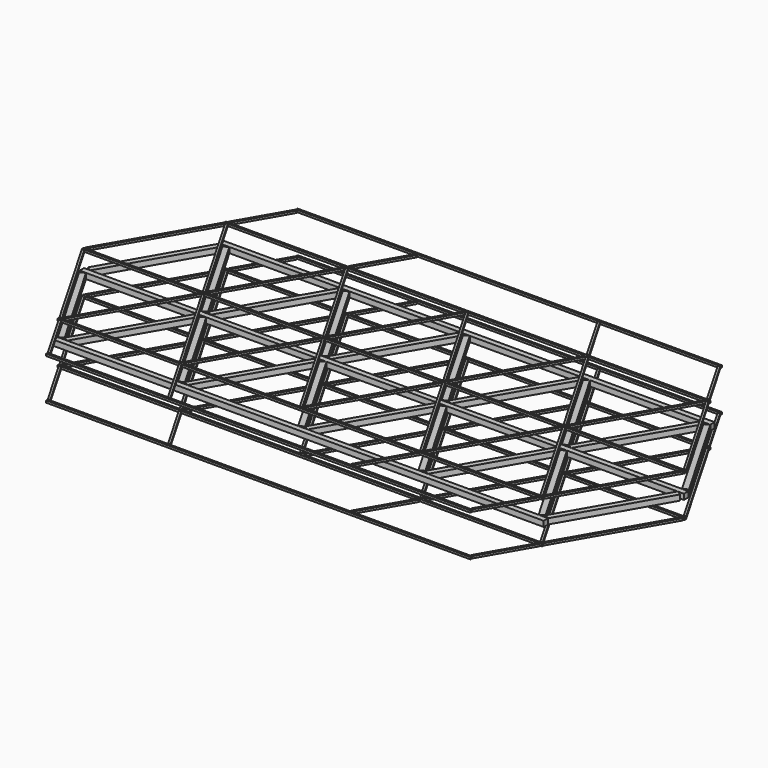
from build123d import *

# Parameters (mm, degrees)
F4_DEPTH = 20
F6_DEPTH = 7.5


# Not quite as in the source:
# - a feature names something its author has since deleted; it is built from what else it names


with BuildPart() as f4:
    # F2 (on Top) → F4 (new body, symmetric)
    with BuildSketch(Plane.XY):
        Polygon((-1789.7858344878, 780), (-1789.7858344878, 740), (-1720.5038021851, 740), (-912.2134253196, 740), (-842.9313930169, 740), (-34.6410161514, 740), (0, 740), (34.6410161514, 740), (842.9313930169, 740), (912.2134253196, 740), (1720.5038021851, 740), (1789.7858344878, 740), (1789.7858344878, 780), (0, 780), align=None)
    extrude(amount=F4_DEPTH, both=True)


with BuildPart() as f4b:
    # F2 (on Top) → F4, piece 2 (new body, symmetric)
    with BuildSketch(Plane.XY):
        Polygon((-2193.9310229206, 40), (-2159.2900067692, 20), (-1755.1448183365, 720), (-1772.4653264122, 730), (-1789.7858344878, 740), align=None)
    extrude(amount=F4_DEPTH, both=True)


with BuildPart() as f4c:
    # F2 (on Top) → F4, piece 3 (new body, symmetric)
    with BuildSketch(Plane.XY):
        Polygon((-1755.1448183365, 720), (-1350.9996299037, 20), (-1333.679121828, 30), (-1316.3586137523, 40), (-1720.5038021851, 740), (-1737.8243102608, 730), align=None)
    extrude(amount=F4_DEPTH, both=True)


with BuildPart() as f4d:
    # F2 (on Top) → F4, piece 4 (new body, symmetric)
    with BuildSketch(Plane.XY):
        Polygon((-1299.0381056767, 30), (-1281.717597601, 20), (-877.5724091682, 720), (-894.8929172439, 730), (-912.2134253196, 740), (-1316.3586137523, 40), align=None)
    extrude(amount=F4_DEPTH, both=True)


with BuildPart() as f4e:
    # F2 (on Top) → F4, piece 5 (new body, symmetric)
    with BuildSketch(Plane.XY):
        Polygon((-877.5724091682, 720), (-473.4272207355, 20), (-456.1067126598, 30), (-438.7862045841, 40), (-842.9313930169, 740), (-860.2519010925, 730), align=None)
    extrude(amount=F4_DEPTH, both=True)


with BuildPart() as f4f:
    # F2 (on Top) → F4, piece 6 (new body, symmetric)
    with BuildSketch(Plane.XY):
        Polygon((-421.4656965084, 30), (-404.1451884327, 20), (0, 720), (-17.3205080757, 730), (-34.6410161514, 740), (-438.7862045841, 40), align=None)
    extrude(amount=F4_DEPTH, both=True)


with BuildPart() as f4g:
    # F2 (on Top) → F4, piece 7 (new body, symmetric)
    with BuildSketch(Plane.XY):
        Polygon((17.3205080757, 730), (0, 720), (404.1451884327, 20), (421.4656965084, 30), (438.7862045841, 40), (34.6410161514, 740), align=None)
    extrude(amount=F4_DEPTH, both=True)


with BuildPart() as f4h:
    # F2 (on Top) → F4, piece 8 (new body, symmetric)
    with BuildSketch(Plane.XY):
        Polygon((456.1067126598, 30), (473.4272207355, 20), (877.5724091682, 720), (860.2519010925, 730), (842.9313930169, 740), (438.7862045841, 40), align=None)
    extrude(amount=F4_DEPTH, both=True)


with BuildPart() as f4i:
    # F2 (on Top) → F4, piece 9 (new body, symmetric)
    with BuildSketch(Plane.XY):
        Polygon((894.8929172439, 730), (877.5724091682, 720), (1281.717597601, 20), (1299.0381056767, 30), (1316.3586137523, 40), (912.2134253196, 740), align=None)
    extrude(amount=F4_DEPTH, both=True)


with BuildPart() as f4j:
    # F2 (on Top) → F4, piece 10 (new body, symmetric)
    with BuildSketch(Plane.XY):
        Polygon((1737.8243102608, 730), (1720.5038021851, 740), (1316.3586137523, 40), (1333.679121828, 30), (1350.9996299037, 20), (1755.1448183365, 720), align=None)
    extrude(amount=F4_DEPTH, both=True)


with BuildPart() as f4k:
    # F2 (on Top) → F4, piece 11 (new body, symmetric)
    with BuildSketch(Plane.XY):
        Polygon((1316.3586137523, -40), (1720.5038021851, -740), (1737.8243102608, -730), (1755.1448183365, -720), (1350.9996299037, -20), (1333.679121828, -30), align=None)
    extrude(amount=F4_DEPTH, both=True)


with BuildPart() as f4l:
    # F2 (on Top) → F4, piece 12 (new body, symmetric)
    with BuildSketch(Plane.XY):
        Polygon((1281.717597601, -20), (877.5724091682, -720), (894.8929172439, -730), (912.2134253196, -740), (1316.3586137523, -40), (1299.0381056767, -30), align=None)
    extrude(amount=F4_DEPTH, both=True)


with BuildPart() as f4m:
    # F2 (on Top) → F4, piece 13 (new body, symmetric)
    with BuildSketch(Plane.XY):
        Polygon((877.5724091682, -720), (473.4272207355, -20), (456.1067126598, -30), (438.7862045841, -40), (842.9313930169, -740), (860.2519010925, -730), align=None)
    extrude(amount=F4_DEPTH, both=True)


with BuildPart() as f4n:
    # F2 (on Top) → F4, piece 14 (new body, symmetric)
    with BuildSketch(Plane.XY):
        Polygon((404.1451884327, -20), (0, -720), (17.3205080757, -730), (34.6410161514, -740), (438.7862045841, -40), (421.4656965084, -30), align=None)
    extrude(amount=F4_DEPTH, both=True)


with BuildPart() as f4o:
    # F2 (on Top) → F4, piece 15 (new body, symmetric)
    with BuildSketch(Plane.XY):
        Polygon((0, -720), (-404.1451884327, -20), (-421.4656965084, -30), (-438.7862045841, -40), (-34.6410161514, -740), (-17.3205080757, -730), align=None)
    extrude(amount=F4_DEPTH, both=True)


with BuildPart() as f4p:
    # F2 (on Top) → F4, piece 16 (new body, symmetric)
    with BuildSketch(Plane.XY):
        Polygon((-456.1067126598, -30), (-473.4272207355, -20), (-877.5724091682, -720), (-860.2519010925, -730), (-842.9313930169, -740), (-438.7862045841, -40), align=None)
    extrude(amount=F4_DEPTH, both=True)


with BuildPart() as f4q:
    # F2 (on Top) → F4, piece 17 (new body, symmetric)
    with BuildSketch(Plane.XY):
        Polygon((-877.5724091682, -720), (-1281.717597601, -20), (-1299.0381056767, -30), (-1316.3586137523, -40), (-912.2134253196, -740), (-894.8929172439, -730), align=None)
    extrude(amount=F4_DEPTH, both=True)


with BuildPart() as f4r:
    # F2 (on Top) → F4, piece 18 (new body, symmetric)
    with BuildSketch(Plane.XY):
        Polygon((-1333.679121828, -30), (-1350.9996299037, -20), (-1755.1448183365, -720), (-1737.8243102608, -730), (-1720.5038021851, -740), (-1316.3586137523, -40), align=None)
    extrude(amount=F4_DEPTH, both=True)


with BuildPart() as f4s:
    # F2 (on Top) → F4, piece 19 (new body, symmetric)
    with BuildSketch(Plane.XY):
        Polygon((-1755.1448183365, -720), (-2159.2900067692, -20), (-2193.9310229206, -40), (-1789.7858344878, -740), (-1772.4653264122, -730), align=None)
    extrude(amount=F4_DEPTH, both=True)


with BuildPart() as f4t:
    # F2 (on Top) → F4, piece 20 (new body, symmetric)
    with BuildSketch(Plane.XY):
        Polygon((-1720.5038021851, -740), (-1789.7858344878, -740), (-1789.7858344878, -780), (0, -780), (1789.7858344878, -780), (1789.7858344878, -740), (1720.5038021851, -740), (912.2134253196, -740), (842.9313930169, -740), (34.6410161514, -740), (0, -740), (-34.6410161514, -740), (-842.9313930169, -740), (-912.2134253196, -740), align=None)
    extrude(amount=F4_DEPTH, both=True)


with BuildPart() as f4u:
    # F2 (on Top) → F4, piece 21 (new body, symmetric)
    with BuildSketch(Plane.XY):
        Polygon((1772.4653264122, -730), (1789.7858344878, -740), (2193.9310229206, -40), (2159.2900067692, -20), (1755.1448183365, -720), align=None)
    extrude(amount=F4_DEPTH, both=True)


with BuildPart() as f4v:
    # F2 (on Top) → F4, piece 22 (new body, symmetric)
    with BuildSketch(Plane.XY):
        Polygon((2193.9310229206, 40), (1789.7858344878, 740), (1772.4653264122, 730), (1755.1448183365, 720), (2159.2900067692, 20), align=None)
    extrude(amount=F4_DEPTH, both=True)


with BuildPart() as f4w:
    # F2 (on Top) → F4, piece 23 (new body, symmetric)
    with BuildSketch(Plane.XY):
        Polygon((-2159.2900067692, 20), (-2205.4780283044, 20), (-2205.4780283044, -20), (-2159.2900067692, -20), (-1350.9996299037, -20), (-1281.717597601, -20), (-473.4272207355, -20), (-404.1451884327, -20), (0, -20), (404.1451884327, -20), (473.4272207355, -20), (1281.717597601, -20), (1350.9996299037, -20), (2159.2900067692, -20), (2205.4780283044, -20), (2205.4780283044, 20), (2159.2900067692, 20), (1350.9996299037, 20), (1281.717597601, 20), (473.4272207355, 20), (404.1451884327, 20), (0, 20), (-404.1451884327, 20), (-473.4272207355, 20), (-1281.717597601, 20), (-1350.9996299037, 20), align=None)
    extrude(amount=F4_DEPTH, both=True)


with BuildPart() as f6:
    # F5 (on offset) → F6 (new body, symmetric)
    with BuildSketch(Plane.XY.offset(150)):
        Polygon((-1329.3489948091, 7.5), (-2180.9406418638, 7.5), (-2198.2611499395, 7.5), (-2198.2611499395, 0), (-2198.2611499395, -7.5), (-2180.9406418638, -7.5), (-1329.3489948091, -7.5), (-1303.3682326956, -7.5), (-451.7765856409, -7.5), (-425.7958235273, -7.5), (0, -7.5), (425.7958235273, -7.5), (451.7765856409, -7.5), (1303.3682326956, -7.5), (1329.3489948091, -7.5), (2180.9406418638, -7.5), (2198.2611499395, -7.5), (2198.2611499395, 0), (2198.2611499395, 7.5), (2180.9406418638, 7.5), (1329.3489948091, 7.5), (1303.3682326956, 7.5), (451.7765856409, 7.5), (425.7958235273, 7.5), (0, 7.5), (-425.7958235273, 7.5), (-451.7765856409, 7.5), (-1303.3682326956, 7.5), align=None)
    extrude(amount=F6_DEPTH, both=True)

    # F5 (on offset) → F6, piece 2 (join, symmetric)
    with BuildSketch(Plane.XY.offset(150)):
        Polygon((-1761.6400088648, 748.75), (-1768.1351993932, 752.5), (-2193.9310229206, 15), (-2187.4358323922, 11.25), (-2180.9406418638, 7.5), (-1755.1448183365, 745), align=None)
    extrude(amount=F6_DEPTH, both=True)

    # F5 (on offset) → F6, piece 3 (join, symmetric)
    with BuildSketch(Plane.XY.offset(150)):
        Polygon((-1316.3586137523, 15), (-1742.1544372797, 752.5), (-1748.6496278081, 748.75), (-1755.1448183365, 745), (-1329.3489948091, 7.5), (-1322.8538042807, 11.25), align=None)
    extrude(amount=F6_DEPTH, both=True)

    # F5 (on offset) → F6, piece 4 (join, symmetric)
    with BuildSketch(Plane.XY.offset(150)):
        Polygon((-884.0675996966, 748.75), (-890.562790225, 752.5), (-1316.3586137523, 15), (-1309.863423224, 11.25), (-1303.3682326956, 7.5), (-877.5724091682, 745), align=None)
    extrude(amount=F6_DEPTH, both=True)

    # F5 (on offset) → F6, piece 5 (join, symmetric)
    with BuildSketch(Plane.XY.offset(150)):
        Polygon((-438.7862045841, 15), (-864.5820281115, 752.5), (-871.0772186398, 748.75), (-877.5724091682, 745), (-451.7765856409, 7.5), (-445.2813951125, 11.25), align=None)
    extrude(amount=F6_DEPTH, both=True)



with BuildPart() as f6b:
    # F5 (on offset) → F6, piece 6 (new body, symmetric)
    with BuildSketch(Plane.XY.offset(150)):
        Polygon((-1535.7517160444, 1125), (-1542.2469065728, 1128.75), (-1548.7420971012, 1132.5), (-1755.1448183365, 775), (-1748.6496278081, 771.25), (-1742.1544372797, 767.5), align=None)
    extrude(amount=F6_DEPTH, both=True)


with BuildPart() as f6_1:
    add(f6.part)

    add(f6b.part)  # F6#7 merges F6b
    # F5 (on offset) → F6, piece 7 (join, symmetric)
    with BuildSketch(Plane.XY.offset(150)):
        Polygon((-864.5820281115, 767.5), (-1742.1544372797, 767.5), (-1768.1351993932, 767.5), (-1768.1351993932, 760), (-1768.1351993932, 752.5), (-1742.1544372797, 752.5), (-890.562790225, 752.5), (-864.5820281115, 752.5), (-12.9903810568, 752.5), (0, 752.5), (12.9903810568, 752.5), (864.5820281115, 752.5), (890.562790225, 752.5), (1742.1544372797, 752.5), (1768.1351993932, 752.5), (1768.1351993932, 760), (1768.1351993932, 767.5), (1742.1544372797, 767.5), (864.5820281115, 767.5), (0, 767.5), align=None)
    extrude(amount=F6_DEPTH, both=True)

    # F5 (on offset) → F6, piece 8 (join, symmetric)
    with BuildSketch(Plane.XY.offset(150)):
        Polygon((-664.6744974046, 1128.75), (-671.1696879329, 1132.5), (-877.5724091682, 775), (-871.0772186398, 771.25), (-864.5820281115, 767.5), (-658.1793068762, 1125), align=None)
    extrude(amount=F6_DEPTH, both=True)

    # F5 (on offset) → F6, piece 9 (join, symmetric)
    with BuildSketch(Plane.XY.offset(150)):
        Polygon((-6.4951905284, 748.75), (-12.9903810568, 752.5), (-438.7862045841, 15), (-432.2910140557, 11.25), (-425.7958235273, 7.5), (0, 745), align=None)
    extrude(amount=F6_DEPTH, both=True)

    # F5 (on offset) → F6, piece 10 (join, symmetric)
    with BuildSketch(Plane.XY.offset(150)):
        Polygon((438.7862045841, 15), (12.9903810568, 752.5), (6.4951905284, 748.75), (0, 745), (425.7958235273, 7.5), (432.2910140557, 11.25), align=None)
    extrude(amount=F6_DEPTH, both=True)

    # F5 (on offset) → F6, piece 11 (join, symmetric)
    with BuildSketch(Plane.XY.offset(150)):
        Polygon((877.5724091682, 775), (671.1696879329, 1132.5), (664.6744974046, 1128.75), (658.1793068762, 1125), (864.5820281115, 767.5), (871.0772186398, 771.25), align=None)
    extrude(amount=F6_DEPTH, both=True)

    # F5 (on offset) → F6, piece 12 (join, symmetric)
    with BuildSketch(Plane.XY.offset(150)):
        Polygon((1755.1448183365, 775), (1548.7420971012, 1132.5), (1542.2469065728, 1128.75), (1535.7517160444, 1125), (1742.1544372797, 767.5), (1748.6496278081, 771.25), align=None)
    extrude(amount=F6_DEPTH, both=True)

    # F5 (on offset) → F6, piece 13 (join, symmetric)
    with BuildSketch(Plane.XY.offset(150)):
        Polygon((1748.6496278081, 748.75), (1742.1544372797, 752.5), (1316.3586137523, 15), (1322.8538042807, 11.25), (1329.3489948091, 7.5), (1755.1448183365, 745), align=None)
    extrude(amount=F6_DEPTH, both=True)

    # F5 (on offset) → F6, piece 14 (join, symmetric)
    with BuildSketch(Plane.XY.offset(150)):
        Polygon((1316.3586137523, 15), (890.562790225, 752.5), (884.0675996966, 748.75), (877.5724091682, 745), (1303.3682326956, 7.5), (1309.863423224, 11.25), align=None)
    extrude(amount=F6_DEPTH, both=True)

    # F5 (on offset) → F6, piece 15 (join, symmetric)
    with BuildSketch(Plane.XY.offset(150)):
        Polygon((871.0772186398, 748.75), (864.5820281115, 752.5), (438.7862045841, 15), (445.2813951125, 11.25), (451.7765856409, 7.5), (877.5724091682, 745), align=None)
    extrude(amount=F6_DEPTH, both=True)

    # F5 (on offset) → F6, piece 16 (join, symmetric)
    with BuildSketch(Plane.XY.offset(150)):
        Polygon((2193.9310229206, 15), (1768.1351993932, 752.5), (1761.6400088648, 748.75), (1755.1448183365, 745), (2180.9406418638, 7.5), (2187.4358323922, 11.25), align=None)
    extrude(amount=F6_DEPTH, both=True)

    # F5 (on offset) → F6, piece 17 (join, symmetric)
    with BuildSketch(Plane.XY.offset(150)):
        Polygon((-1548.7420971012, 1140), (-1548.7420971012, 1132.5), (-671.1696879329, 1132.5), (0, 1132.5), (0, 1140), (0, 1147.5), (-1548.7420971012, 1147.5), align=None)
        Polygon((0, 1140), (0, 1132.5), (671.1696879329, 1132.5), (1548.7420971012, 1132.5), (1548.7420971012, 1140), (1548.7420971012, 1147.5), (0, 1147.5), align=None)
    extrude(amount=F6_DEPTH, both=True)

    # F7: F6 across plane


with BuildPart() as f6_2:
    add(f6_1.part)
    add(f6_1.part.mirror(Plane.XZ))


with BuildPart() as f8_1:
    # F8: instance of F6
    add(f6_2.part.mirror(Plane.XY))


solid = Compound([f4.part, f4b.part, f4c.part, f4d.part, f4e.part, f4f.part, f4g.part, f4h.part, f4i.part, f4j.part, f4k.part, f4l.part, f4m.part, f4n.part, f4o.part, f4p.part, f4q.part, f4r.part, f4s.part, f4t.part, f4u.part, f4v.part, f4w.part, f6_2.part, f8_1.part])
